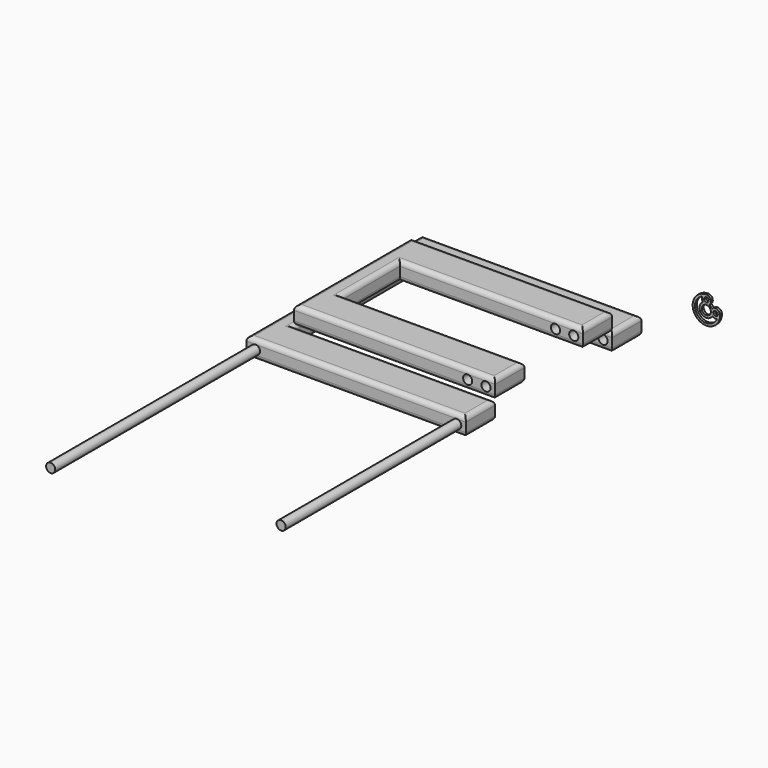
from build123d import *

# Parameters (mm, degrees)
F0_W      = 304.8
F0_H      = 25.4
F0_R      = 6.35
F1_DEPTH  = 304.8
F3_DEPTH  = 25.4
F4_R      = 6.35
F5_DEPTH  = 254.001
F2_W      = 254
F2_H      = 101.6
F6_DEPTH  = 25.401
F7_R      = 6.35
F8_DEPTH  = 304.8
F9_R      = 6.35
F10_DEPTH = 355.6
F11_R     = 6.34999
F11_2_R   = 6.34999
F14_DEPTH = 3.175


# Not quite as in the source:
# - a fillet or chamfer is up to 0.001 mm smaller than in the source, because OpenCascade refuses the exact size
# - a feature names something its author has since deleted; it is built from what else it names


with BuildPart() as f1:
    # F0 (on Front) → F1 (new body)
    with BuildSketch(Plane.XZ):
        with Locations((-152.4, 12.7)):
            Rectangle(F0_W, F0_H)
        with Locations((-292.1, 12.7)):
            Circle(F0_R, mode=Mode.SUBTRACT)
        with Locations((-12.7, 12.7)):
            Circle(F0_R, mode=Mode.SUBTRACT)
    extrude(amount=F1_DEPTH)

    # F2 (on face) → F6 (cut, through all)
    with BuildSketch(Plane.XY.offset(25.4)):
        Polygon((0, -101.6), (0, -50.8), (-279.4, -50.8), (-279.4, -254), (0, -254), (0, -203.2), (-254, -203.2), (-254, -101.6), align=None)
        with Locations((-127, -152.4)):
            Rectangle(F2_W, F2_H)
    extrude(amount=-F6_DEPTH, mode=Mode.SUBTRACT)

    # F11 (radius 6.35 in the source; OpenCascade refuses exactly that, so slightly less here)
    f11_edges = [f1.edges().sort_by_distance(p)[0] for p in [
        (-152.4, 0, 25.4),
        (-304.8, -152.4, 25.4),
        (-152.4, -304.8, 25.4),
        (0, -279.4, 25.4),
        (-139.7, -254, 25.4),
        (-279.4, -152.4, 25.4),
        (-139.7, -50.8, 25.4),
        (0, -25.4, 25.4),
        (-152.4, 0, 0),
        (0, -25.4, 0),
        (-139.7, -50.8, 0),
        (-279.4, -152.4, 0),
        (-139.7, -254, 0),
        (0, -279.4, 0),
        (-152.4, -304.8, 0),
        (-304.8, -152.4, 0),
    ]]
    fillet(f11_edges, radius=F11_R)


with BuildPart() as f3:
    # F2 (on face) → F3 (new body)
    with BuildSketch(Plane.XY.offset(25.4)):
        Polygon((0, -101.6), (0, -50.8), (-279.4, -50.8), (-279.4, -254), (0, -254), (0, -203.2), (-254, -203.2), (-254, -101.6), align=None)
    extrude(amount=F3_DEPTH)

    # F4 (on face) → F5 (cut, through all)
    with BuildSketch(Plane(origin=(0, -50.8, 0), x_dir=(-1, 0, 0), z_dir=(0, 1, 0))):
        with Locations((12.7, 38.1)):
            Circle(F4_R)
        with Locations((38.1, 38.1)):
            Circle(F4_R)
    extrude(amount=-F5_DEPTH, mode=Mode.SUBTRACT)

    # F11#2 (radius 6.35 in the source; OpenCascade refuses exactly that, so slightly less here)
    f11_2_edges = [f3.edges().sort_by_distance(p)[0] for p in [
        (-139.7, -254, 25.4),
        (-279.4, -152.4, 25.4),
        (-139.7, -50.8, 25.4),
        (0, -76.2, 50.8),
        (-139.7, -50.8, 50.8),
        (-279.4, -152.4, 50.8),
        (-139.7, -254, 50.8),
        (0, -228.6, 50.8),
        (-127, -203.2, 50.8),
        (-254, -152.4, 50.8),
        (-127, -101.6, 50.8),
        (0, -76.2, 25.4),
        (0, -228.6, 25.4),
        (-127, -203.2, 25.4),
        (-254, -152.4, 25.4),
        (-127, -101.6, 25.4),
    ]]
    fillet(f11_2_edges, radius=F11_2_R)


with BuildPart() as f8:
    # F7 (on face) → F8 (new body)
    with BuildSketch(Plane.XZ.offset(304.8)):
        with Locations((-12.7, 12.7)):
            Circle(F7_R)
    extrude(amount=F8_DEPTH)


with BuildPart() as f10:
    # F9 (on face) → F10 (new body)
    with BuildSketch(Plane.XZ.offset(304.8)):
        with Locations((-292.1, 12.7)):
            Circle(F9_R)
    extrude(amount=F10_DEPTH)


with BuildPart() as f14:
    # F13 (on offset) → F14 (new body)
    with BuildSketch(Plane.XZ.offset(-152.4)):
        with BuildLine():
            ThreePointArc((-29.2250082641, -18.9096650779), (-42.6953924457, -51.4300492595), (-10.1750082641, -37.9596650779))
            ThreePointArc((-10.1750082641, -37.9596650779), (-11.3809203347, -41.6826825873), (-14.5406332641, -43.9916428514))
            ThreePointArc((-14.5406332641, -43.9916428514), (-40.4503284154, -49.1849852293), (-35.2569860376, -23.2752900779))
            ThreePointArc((-35.2569860376, -23.2752900779), (-32.9480257735, -20.1155771486), (-29.2250082641, -18.9096650779))
        make_face()
        with BuildLine():
            ThreePointArc((-20.8906332641, -42.5709358745), (-22.3578557141, -40.4697229707), (-22.8750082641, -37.9596650779))
            ThreePointArc((-22.8750082641, -37.9596650779), (-33.7151363246, -42.4497931385), (-29.2250082641, -31.6096650779))
            ThreePointArc((-29.2250082641, -31.6096650779), (-31.7350661569, -31.0925125279), (-33.8362790607, -29.6252900779))
            ThreePointArc((-33.8362790607, -29.6252900779), (-35.9602003549, -44.6948571687), (-20.8906332641, -42.5709358745))
        make_face()
        with BuildLine():
            ThreePointArc((-35.2569860376, -23.2752900779), (-35.4218066335, -26.6460957358), (-33.8362790607, -29.6252900779))
            ThreePointArc((-33.8362790607, -29.6252900779), (-31.6062582641, -28.7371234848), (-29.2250082641, -28.4346650779))
            ThreePointArc((-29.2250082641, -28.4346650779), (-32.4000082641, -25.2596650779), (-29.2250082641, -22.0846650779))
            ThreePointArc((-29.2250082641, -22.0846650779), (-32.2991887952, -22.3851654371), (-35.2569860376, -23.2752900779))
        make_face()
        with BuildLine():
            ThreePointArc((-33.8362790607, -29.6252900779), (-31.7350661569, -31.0925125279), (-29.2250082641, -31.6096650779))
            ThreePointArc((-29.2250082641, -31.6096650779), (-26.8833074573, -31.1621168847), (-24.8716929388, -29.8825587257))
            ThreePointArc((-24.8716929388, -29.8825587257), (-23.3955120459, -27.7774962562), (-22.8750082641, -25.2596650779))
            ThreePointArc((-22.8750082641, -25.2596650779), (-24.7348802036, -20.7695370174), (-29.2250082641, -18.9096650779))
            ThreePointArc((-29.2250082641, -18.9096650779), (-32.9480257735, -20.1155771486), (-35.2569860376, -23.2752900779))
            ThreePointArc((-35.2569860376, -23.2752900779), (-32.2991887952, -22.3851654371), (-29.2250082641, -22.0846650779))
            ThreePointArc((-29.2250082641, -22.0846650779), (-26.9799442338, -23.0146010477), (-26.0500082641, -25.2596650779))
            ThreePointArc((-26.0500082641, -25.2596650779), (-26.9799442338, -27.5047291082), (-29.2250082641, -28.4346650779))
            ThreePointArc((-29.2250082641, -28.4346650779), (-31.6062582641, -28.7371234848), (-33.8362790607, -29.6252900779))
        make_face()
        with BuildLine():
            ThreePointArc((-21.1479019119, -33.6063497526), (-22.4274600709, -35.6179642712), (-22.8750082641, -37.9596650779))
            ThreePointArc((-22.8750082641, -37.9596650779), (-22.3578557141, -40.4697229707), (-20.8906332641, -42.5709358745))
            ThreePointArc((-20.8906332641, -42.5709358745), (-20.0024666709, -40.3409150779), (-19.7000082641, -37.9596650779))
            ThreePointArc((-19.7000082641, -37.9596650779), (-16.5250082641, -34.7846650779), (-13.3500082641, -37.9596650779))
            ThreePointArc((-13.3500082641, -37.9596650779), (-13.6505086233, -41.033845609), (-14.5406332641, -43.9916428514))
            ThreePointArc((-14.5406332641, -43.9916428514), (-11.3809203347, -41.6826825873), (-10.1750082641, -37.9596650779))
            ThreePointArc((-10.1750082641, -37.9596650779), (-14.1833074573, -32.0572132711), (-21.1479019119, -33.6063497526))
        make_face()
        with BuildLine():
            ThreePointArc((-19.7000082641, -37.9596650779), (-20.0024666709, -40.3409150779), (-20.8906332641, -42.5709358745))
            ThreePointArc((-20.8906332641, -42.5709358745), (-17.911438922, -44.1564634473), (-14.5406332641, -43.9916428514))
            ThreePointArc((-14.5406332641, -43.9916428514), (-13.6505086233, -41.033845609), (-13.3500082641, -37.9596650779))
            ThreePointArc((-13.3500082641, -37.9596650779), (-16.5250082641, -41.1346650779), (-19.7000082641, -37.9596650779))
        make_face()
        with BuildLine():
            ThreePointArc((-29.2250082641, -31.6096650779), (-24.7348802036, -33.4695370174), (-22.8750082641, -37.9596650779))
            ThreePointArc((-22.8750082641, -37.9596650779), (-22.4274600709, -35.6179642712), (-21.1479019119, -33.6063497526))
            Line((-21.1479019119, -33.6063497526), (-24.8716929388, -29.8825587257))
            ThreePointArc((-24.8716929388, -29.8825587257), (-26.8833074573, -31.1621168847), (-29.2250082641, -31.6096650779))
        make_face()
    extrude(amount=F14_DEPTH)


solid = Compound([f1.part, f3.part, f8.part, f10.part, f14.part])
